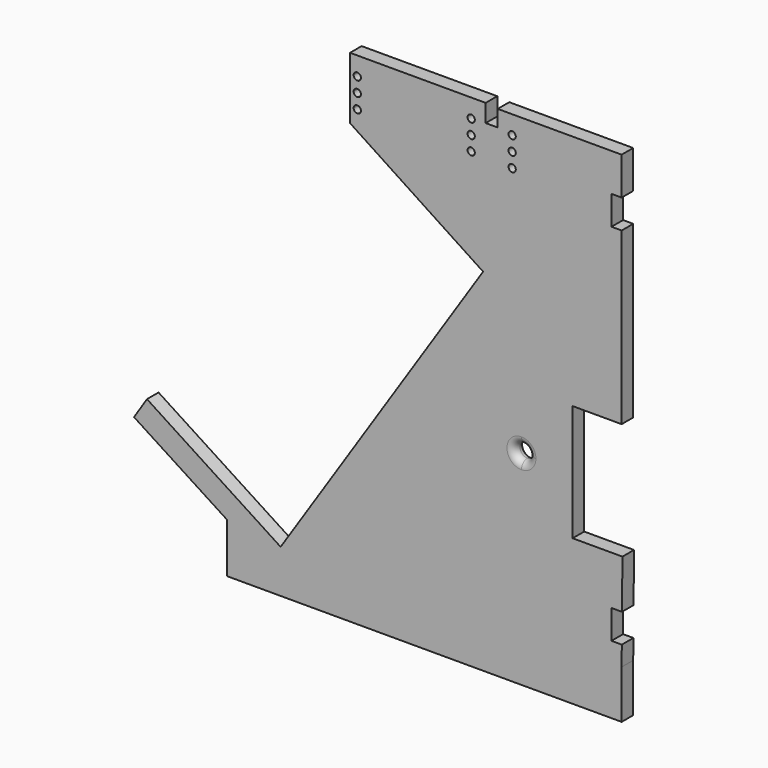
from build123d import *

# Parameters (mm, degrees)
F0_R     = 0.635
F1_DEPTH = 2.54
F2_R     = 1.26999


# Not quite as in the source:
# - a fillet or chamfer is up to 0.001 mm smaller than in the source, because OpenCascade refuses the exact size


with BuildPart() as f1:
    # F0 (on Front) → F1 (new body)
    with BuildSketch(Plane.XZ):
        Polygon((15.0977487051, 33.894000689), (-8.7011743405, 33.894000689), (-8.7011743405, 30.6449289119), (-8.7011743405, 30.6394077664), (-8.7011743405, 28.5887729555), (-8.7011743405, 28.1049289119), (-8.7011743405, 23.0249289119), (21.375445649, 23.0249289119), (37.1712256595, 23.0249289119), (37.1712256595, 27.0205680281), (38.9492256595, 27.0205680281), (38.9492256595, 30.7752811804), (38.9492256595, 33.6518122062), (17.204430995, 33.6518122062), (17.204430995, 30.7752811804), (15.0977487051, 30.7752811804), align=None)
        with BuildLine():
            ThreePointArc((-6.7956986329, 25.5649289119), (-6.9816858268, 25.1159161058), (-7.4306986329, 24.9299289119))
            ThreePointArc((-7.4306986329, 24.9299289119), (-7.8797114389, 25.1159161058), (-8.0656986329, 25.5649289119))
            ThreePointArc((-8.0656986329, 25.5649289119), (-7.8797114389, 26.0139417179), (-7.4306986329, 26.1999289119))
            ThreePointArc((-7.4306986329, 26.1999289119), (-6.9816858268, 26.0139417179), (-6.7956986329, 25.5649289119))
        make_face(mode=Mode.SUBTRACT)
        with BuildLine():
            ThreePointArc((-7.4306986329, 28.7399289119), (-6.9816858268, 28.5539417179), (-6.7956986329, 28.1049289119))
            ThreePointArc((-6.7956986329, 28.1049289119), (-6.9816858268, 27.6559161058), (-7.4306986329, 27.4699289119))
            ThreePointArc((-7.4306986329, 27.4699289119), (-7.8797114389, 27.6559161058), (-8.0656986329, 28.1049289119))
            ThreePointArc((-8.0656986329, 28.1049289119), (-7.8797114389, 28.5539417179), (-7.4306986329, 28.7399289119))
        make_face(mode=Mode.SUBTRACT)
        with BuildLine():
            ThreePointArc((-7.4306986329, 30.0099289119), (-7.8797114389, 30.1959161058), (-8.0656986329, 30.6449289119))
            ThreePointArc((-8.0656986329, 30.6449289119), (-7.8797114389, 31.0939417179), (-7.4306986329, 31.2799289119))
            ThreePointArc((-7.4306986329, 31.2799289119), (-6.9816858268, 31.0939417179), (-6.7956986329, 30.6449289119))
            ThreePointArc((-6.7956986329, 30.6449289119), (-6.9816858268, 30.1959161058), (-7.4306986329, 30.0099289119))
        make_face(mode=Mode.SUBTRACT)
        with BuildLine():
            ThreePointArc((13.1927487051, 25.5649289119), (13.0067615112, 25.1159161058), (12.5577487051, 24.9299289119))
            ThreePointArc((12.5577487051, 24.9299289119), (11.9227487051, 25.5649289119), (12.5577487051, 26.1999289119))
            ThreePointArc((12.5577487051, 26.1999289119), (13.0067615112, 26.0139417179), (13.1927487051, 25.5649289119))
        make_face(mode=Mode.SUBTRACT)
        with BuildLine():
            ThreePointArc((12.5577487051, 28.7399289119), (13.0067615112, 28.5539417179), (13.1927487051, 28.1049289119))
            ThreePointArc((13.1927487051, 28.1049289119), (13.0067615112, 27.6559161058), (12.5577487051, 27.4699289119))
            ThreePointArc((12.5577487051, 27.4699289119), (11.9227487051, 28.1049289119), (12.5577487051, 28.7399289119))
        make_face(mode=Mode.SUBTRACT)
        with BuildLine():
            ThreePointArc((13.1927487051, 30.6449289119), (13.0067615112, 30.1959161058), (12.5577487051, 30.0099289119))
            ThreePointArc((12.5577487051, 30.0099289119), (11.9227487051, 30.6449289119), (12.5577487051, 31.2799289119))
            ThreePointArc((12.5577487051, 31.2799289119), (13.0067615112, 31.0939417179), (13.1927487051, 30.6449289119))
        make_face(mode=Mode.SUBTRACT)
        with Locations((19.744430995, 25.3227458062)):
            Circle(F0_R, mode=Mode.SUBTRACT)
        with Locations((19.744430995, 27.8627458062)):
            Circle(F0_R, mode=Mode.SUBTRACT)
        with Locations((19.744430995, 30.4027458062)):
            Circle(F0_R, mode=Mode.SUBTRACT)
        with BuildLine():
            Line((21.375445649, 23.0249289119), (-8.7011743405, 23.0249289119))
            Line((-8.7011743405, 23.0249289119), (14.6481524707, 7.6804661495))
            Line((14.6481524707, 7.6804661495), (4.3133735196, -8.0457365195))
            Line((4.3133735196, -8.0457365195), (4.3133735196, -53.9590548808))
            Line((4.3133735196, -53.9590548808), (21.375445649, -53.9590548808))
            Line((21.375445649, -53.9590548808), (21.375445649, -19.4510648049))
            ThreePointArc((21.375445649, -19.4510648049), (20.105445649, -18.1810648049), (21.375445649, -16.9110648049))
            Line((21.375445649, -16.9110648049), (21.375445649, 23.0249289119))
        make_face()
        with BuildLine():
            Line((37.1712256595, 23.0249289119), (21.375445649, 23.0249289119))
            Line((21.375445649, 23.0249289119), (21.375445649, -16.9110648049))
            ThreePointArc((21.375445649, -16.9110648049), (22.2734712611, -17.2830391928), (22.645445649, -18.1810648049))
            Line((22.645445649, -18.1810648049), (30.3538220114, -18.1810648049))
            Line((30.3538220114, -18.1810648049), (30.3538220114, -7.9758184713))
            Line((30.3538220114, -7.9758184713), (38.9492256595, -7.9758184713))
            Line((38.9492256595, -7.9758184713), (38.9492256595, 5.319000689))
            Line((38.9492256595, 5.319000689), (38.9492256595, 21.9405680281))
            Line((38.9492256595, 21.9405680281), (37.1712256595, 21.9405680281))
            Line((37.1712256595, 21.9405680281), (37.1712256595, 23.0249289119))
        make_face()
        Polygon((4.3133735196, -53.9590548808), (4.3133735196, -8.0457365195), (-20.8784960799, -46.3796427219), (-44.3256125721, -31.185070223), (-46.598433602, -34.7022139158), (-30.3224786203, -45.2199339734), (-30.3224786203, -53.9590548808), align=None)
        with BuildLine():
            Line((30.3538220114, -18.1810648049), (22.645445649, -18.1810648049))
            ThreePointArc((22.645445649, -18.1810648049), (22.2734712611, -19.079090417), (21.375445649, -19.4510648049))
            Line((21.375445649, -19.4510648049), (21.375445649, -53.9590548808))
            Line((21.375445649, -53.9590548808), (38.9492256595, -53.9590548808))
            Line((38.9492256595, -53.9590548808), (38.9492256595, -45.480999311))
            Line((38.9492256595, -45.480999311), (38.9492256595, -42.0136552247))
            Line((38.9492256595, -42.0136552247), (37.1712256595, -42.0136552247))
            Line((37.1712256595, -42.0136552247), (37.1712256595, -36.9336552247))
            Line((37.1712256595, -36.9336552247), (38.9492256595, -36.9336552247))
            Line((38.9492256595, -36.9336552247), (38.9492256595, -28.3863111384))
            Line((38.9492256595, -28.3863111384), (30.3538220114, -28.3863111384))
            Line((30.3538220114, -28.3863111384), (30.3538220114, -18.1810648049))
        make_face()
        Polygon((38.9492256595, -42.0136552247), (38.9492256595, -45.480999311), (38.9764610146, -42.0136552247), align=None)
        Polygon((39.0835013158, -28.3863111384), (38.9492256595, -28.3863111384), (38.9492256595, -36.9336552247), (39.0163634877, -36.9336552247), align=None)
    extrude(amount=F1_DEPTH)

    # F2 (radius 1.27 in the source; OpenCascade refuses exactly that, so slightly less here)
    f2_edges = [f1.edges().sort_by_distance(p)[0] for p in [
        (20.105446, -2.54, -18.181065),
        (20.105446, 0, -18.181065),
    ]]
    fillet(f2_edges, radius=F2_R)


solid = f1.part
